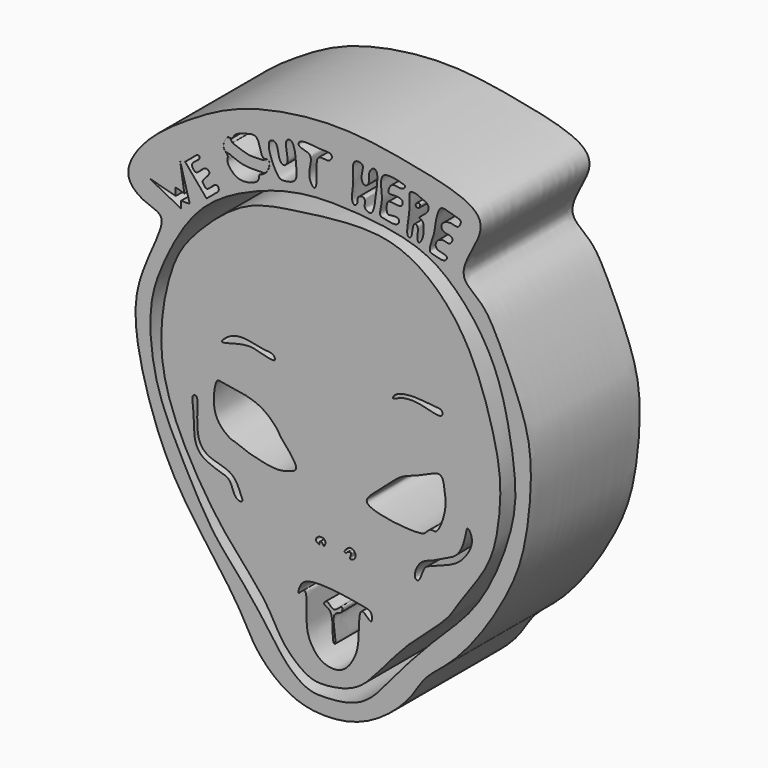
from build123d import *

# Parameters (mm, degrees)
F1_DEPTH = 12


# Not quite as in the source:
# - a feature names something its author has since deleted; it is built from what else it names


with BuildPart() as f1:
    # F0 (on Front) → F1 (new body)
    with BuildSketch(Plane.XZ):
        with BuildLine():
            add(Edge.make_bspline(
                [(-47.0166243613, 44.8620691895), (-45.595251877, 45.776944077), (-42.2741227464, 47.7877491265), (-34.0176381654, 49.1391279437), (-27.6370435065, 48.027277594), (-23.191439719, 47.1215840657), (-21.197445005, 46.0254771062), (-20.9193717284, 44.4684259144), (-22.5035572971, 42.0546528765), (-22.7690901071, 40.3377748917), (-20.8843213118, 39.2071538838), (-19.6447559897, 37.0583489704), (-17.633566432, 32.6179743092), (-16.4023527537, 28.7667152956), (-16.916817699, 22.3336429781), (-18.0728468976, 18.3576353556), (-20.7470243169, 13.731212027), (-23.6453545353, 10.2470769915), (-26.1614221001, 8.5326667329), (-27.2405305623, 6.2194756967), (-30.5742150796, 3.3267319265), (-34.1911424438, 2.4165036843), (-37.8655474923, 2.8581800799), (-40.9480017394, 5.5727937583), (-42.1845902774, 8.3976566392), (-45.0170046598, 12.252109148), (-47.5829757261, 15.6966068437), (-49.6990101842, 19.8737084463), (-51.4091567908, 25.4811818071), (-51.8436489228, 30.6040680499), (-49.3464398381, 35.1945462838), (-49.0787891391, 36.9579414452), (-50.8399233715, 37.2709356223), (-52.8928865029, 38.9279900141), (-50.646604664, 42.436379878), (-48.3189845132, 44.0237973006), (-47.0166243613, 44.8620691895)],
                knots=[0, 0, 0, 0, 0.0355770683, 0.0793528757, 0.1187531848, 0.1509720013, 0.1725011929, 0.1899685641, 0.2157418654, 0.2344161387, 0.2552668169, 0.2794632534, 0.3127171361, 0.3440503941, 0.3820044117, 0.4134842243, 0.4484589959, 0.4811195553, 0.5068947662, 0.5308536817, 0.5623016146, 0.5916301045, 0.620359809, 0.6502239744, 0.6771282332, 0.7101499943, 0.7419335424, 0.7747889469, 0.8115699797, 0.8464105758, 0.8808110455, 0.8982397629, 0.9169922383, 0.93908403, 0.96740182, 1, 1, 1, 1], degree=3))
        make_face()
        with BuildLine():
            add(Edge.make_bspline(
                [(-38.4240150452, 42.1812050045), (-37.0678788492, 42.5218744662), (-34.3867781007, 42.8088010896), (-28.3798473119, 42.3274214714), (-24.1902437, 40.8098863437), (-19.8961635432, 35.6901117013), (-18.6253817253, 30.528621672), (-18.0581329266, 27.0595758172), (-17.8633858275, 23.0739012141), (-20.7079995076, 15.7863490066), (-24.450016641, 12.3873464297), (-27.2230581422, 9.3965022394), (-29.0126764634, 7.3723433058), (-31.2995555124, 4.3586146755), (-34.6274425345, 4.0112345038), (-36.4516832364, 4.0578458846), (-38.3722620753, 5.6080571102), (-39.6856518206, 7.5759460913), (-42.1423981818, 10.8035289735), (-44.8206668482, 13.5361271115), (-47.6013889681, 18.7964344106), (-49.9213569734, 23.4284872311), (-50.5031038055, 29.324048), (-49.2168686424, 33.0878991596), (-46.6874092768, 37.918528947), (-43.0773019309, 40.6065854083), (-39.8897478434, 41.8130042257), (-38.4240150452, 42.1812050045)],
                knots=[0, 0, 0, 0, 0.0393324741, 0.0861492727, 0.1269776985, 0.1760073002, 0.2206521584, 0.2561939723, 0.2945424829, 0.3480010505, 0.3922375976, 0.4304492998, 0.4625965925, 0.4993837574, 0.5337407214, 0.5595497864, 0.5886036071, 0.6188415895, 0.6572680082, 0.6956866915, 0.7423767025, 0.7873017999, 0.8331769589, 0.8719791181, 0.9163532505, 0.9574888588, 1, 1, 1, 1], degree=3))
        make_face(mode=Mode.SUBTRACT)
        Polygon((-47.5117638707, 37.8683283925), (-50.2995289862, 39.3151417375), (-47.9881539941, 38.6976003647), (-47.9881539941, 39.3680743873), (-47.2294613719, 39.1387008131), (-47.5999861956, 41.5382944047), (-46.7530712485, 38.4858697653), (-47.5117638707, 38.4858697653), align=None, mode=Mode.SUBTRACT)
        with BuildLine():
            Line((-45.2709682286, 39.3857210875), (-47.1588820219, 41.6265167296))
            Line((-47.1588820219, 41.6265167296), (-46.1392381304, 42.4855864863))
            add(Edge.make_bspline(
                [(-46.1392381304, 42.4855864863), (-46.0465615658, 42.5054674734), (-45.8594185494, 42.5456134145), (-45.8520416375, 42.1577943123), (-46.6511050845, 41.7832702106), (-46.4903258591, 41.2952470764), (-46.1022131536, 40.9477511118), (-45.5256395853, 41.8046746664), (-45.067552008, 41.6403244999), (-44.9381597234, 41.3477459308), (-45.6719466599, 40.6847546609), (-45.5906592697, 40.4745039867), (-45.1946911115, 39.8798795628), (-44.5937516593, 40.8455123959), (-44.1630185636, 40.6303502121), (-44.1921356311, 40.3988699414), (-44.2067978835, 40.282305245)],
                knots=[0, 0, 0, 0, 0.052085804, 0.105177555, 0.2008801244, 0.2698978457, 0.3346360985, 0.4345195347, 0.5005230921, 0.55286709, 0.6548123539, 0.7045411848, 0.7779620534, 0.8784844899, 0.9388093918, 1, 1, 1, 1], degree=3))
            Line((-44.2067978835, 40.282305245), (-45.2709682286, 39.3857210875))
        make_face(mode=Mode.SUBTRACT)
        with BuildLine():
            add(Edge.make_bspline(
                [(-43.2456322014, 44.7879135609), (-43.1773507865, 44.7833628103), (-43.1203474246, 44.7420608165), (-43.0675894022, 44.7582378983)],
                knots=[0.9714162948, 0.9714162948, 0.9714162948, 0.9714162948, 1, 1, 1, 1], degree=3))
            add(Edge.make_bspline(
                [(-43.0675894022, 44.7582378983), (-42.9989112357, 44.7792965406), (-42.8691053132, 45.0293929425), (-42.6221246051, 45.3184155301), (-41.7475783885, 45.5732360318), (-40.5945532549, 45.8870759647), (-40.4806599693, 43.8436857931), (-39.9417733644, 44.2096012545), (-39.8331619799, 44.1647656262)],
                knots=[0, 0, 0, 0, 0.0372090608, 0.0785561522, 0.1434088997, 0.2074830467, 0.2888642065, 0.3329958717, 0.3329958717, 0.3329958717, 0.3329958717], degree=3))
            add(Edge.make_bspline(
                [(-39.8331619538, 44.1647656213), (-39.7602766999, 44.151206379), (-39.7284395126, 44.0661324711), (-39.7243966212, 43.9518775136)],
                knots=[0.2945540531, 0.2945540531, 0.2945540531, 0.2945540531, 0.3190794148, 0.3190794148, 0.3190794148, 0.3190794148], degree=3))
            add(Edge.make_bspline(
                [(-39.7243966212, 43.9518775136), (-39.7113465111, 43.832177882), (-39.7669607284, 43.3489257107), (-40.2487411874, 42.8370991823), (-40.6788729245, 42.8083932279), (-40.6142458833, 42.3132435515), (-41.0418230498, 41.9490622949), (-42.1032965277, 41.6892524188), (-42.908668964, 42.0081766665), (-43.5614733789, 42.8371202287), (-43.2981182226, 43.3150401101), (-43.5696992665, 43.5194752336), (-43.660394971, 43.6435321849)],
                knots=[0.3580242307, 0.3580242307, 0.3580242307, 0.3580242307, 0.3862259474, 0.4480160925, 0.4867681426, 0.5281473049, 0.5763905528, 0.6452541069, 0.7081336536, 0.7733064754, 0.8182050994, 0.8561222233, 0.8561222233, 0.8561222233, 0.8561222233], degree=3))
            add(Edge.make_bspline(
                [(-43.660394971, 43.6435321849), (-43.7865917542, 43.7698978255), (-43.8055004646, 44.0023963662), (-43.7281247793, 44.2474911359)],
                knots=[0.8330439372, 0.8330439372, 0.8330439372, 0.8330439372, 0.8755337844, 0.8755337844, 0.8755337844, 0.8755337844], degree=3))
            add(Edge.make_bspline(
                [(-43.7281247647, 44.2474911871), (-43.6928008455, 44.3719700456), (-43.6167159272, 44.5325123333), (-43.5244744487, 44.6411680027), (-43.4995404875, 44.6661314575)],
                knots=[0.9030772587, 0.9030772587, 0.9030772587, 0.9030772587, 0.9295678201, 0.9390671556, 0.9390671556, 0.9390671556, 0.9390671556], degree=3))
            add(Edge.make_bspline(
                [(-43.4995404875, 44.6661314575), (-43.413944485, 44.7634769709), (-43.3218092162, 44.8182348636), (-43.2456322014, 44.7879135609)],
                knots=[0.9021251558, 0.9021251558, 0.9021251558, 0.9021251558, 0.9263325769, 0.9263325769, 0.9263325769, 0.9263325769], degree=3))
        make_face(mode=Mode.SUBTRACT)
        with BuildLine():
            add(Edge.make_bspline(
                [(-39.7415310144, 45.5790273845), (-39.9445700993, 45.0899409234), (-39.076085851, 43.0825175549), (-38.545065207, 42.9345275653), (-37.3027436398, 43.1510735203), (-37.3185511717, 44.2461944438), (-37.5140119737, 46.4624062707), (-38.2487786003, 46.3009786949), (-38.293273575, 45.7319646594), (-38.1168506677, 44.9346337394), (-38.1015809471, 44.4595086479), (-38.4929023876, 44.0319639145), (-38.9845528625, 44.6133548632), (-38.9777428469, 45.9043106405), (-39.6454047044, 45.8105792398), (-39.7415310144, 45.5790273845)],
                knots=[0, 0, 0, 0, 0.1312235203, 0.1949314617, 0.2786049754, 0.3642703204, 0.4835971299, 0.5359197008, 0.5955830633, 0.6724402957, 0.7304539966, 0.7835419666, 0.8478830825, 0.937873869, 1, 1, 1, 1], degree=3))
        make_face(mode=Mode.SUBTRACT)
        with BuildLine():
            add(Edge.make_bspline(
                [(-37.0067022741, 46.4965216815), (-37.1571867188, 46.4032603575), (-37.2607087523, 45.9546746534), (-35.8664058245, 45.9719520528), (-36.2034844106, 44.6782350919), (-36.2534624056, 43.8823964905), (-35.7949926392, 43.1371333176), (-35.5293838928, 43.6181235302), (-35.6002153106, 44.6731321226), (-35.5539823511, 45.8598584987), (-35.0234132886, 45.8590436672), (-34.4226287785, 45.7488078966), (-34.1439951194, 46.1976469241), (-34.3890364819, 46.5292450078), (-35.2685805871, 46.416806358), (-36.6860703352, 46.6952303203), (-37.0067022741, 46.4965216815)],
                knots=[0, 0, 0, 0, 0.0521113404, 0.1354071728, 0.2208503286, 0.3017367921, 0.3683065166, 0.4148283754, 0.5059676652, 0.5926154433, 0.6458894091, 0.7103345129, 0.7641496111, 0.8087478712, 0.8889681911, 1, 1, 1, 1], degree=3))
        make_face(mode=Mode.SUBTRACT)
        with BuildLine():
            add(Edge.make_bspline(
                [(-32.207518816, 46.4965216815), (-32.4701286429, 46.2505183013), (-32.173270173, 44.9124336744), (-32.5962911284, 43.5742952887), (-32.1932073961, 42.9676291969), (-31.8929098487, 43.4543410085), (-31.996544244, 43.8961039159), (-31.5094488704, 44.0397093737), (-31.2521699762, 43.8771410453), (-31.3619723855, 43.3056399132), (-31.2590036508, 43.0726525174), (-30.7426859742, 42.8393878073), (-30.4429532561, 43.4965999427), (-30.3413501835, 44.6178538877), (-30.0945805073, 46.2277720064), (-30.5166045943, 46.6143201902), (-31.0577042812, 46.1268052258), (-30.8541406305, 45.1759822328), (-31.2721103899, 44.8820149808), (-31.627975952, 45.1482875767), (-31.5915898163, 45.8325901117), (-31.3387005167, 46.6151939086), (-32.0355516895, 46.657614261), (-32.207518816, 46.4965216815)],
                knots=[0, 0, 0, 0, 0.0751043617, 0.1497401555, 0.1896895528, 0.2277881385, 0.2668540958, 0.3051825112, 0.335001314, 0.3792866057, 0.4098807216, 0.4495249579, 0.4945890761, 0.5626496753, 0.6393918126, 0.6760162216, 0.7211153381, 0.7795538627, 0.8162648223, 0.8511361484, 0.9016374869, 0.9508187435, 1, 1, 1, 1], degree=3))
        make_face(mode=Mode.SUBTRACT)
        with BuildLine():
            add(Edge.make_bspline(
                [(-29.6667721123, 46.2495014071), (-30.0210563778, 45.96228624), (-29.6812809427, 44.4997162614), (-29.93374072, 43.6192435306), (-30.016369393, 42.9674318885), (-29.5685790665, 42.9306325776), (-28.6907209596, 42.6813379227), (-28.2151086076, 42.9880501216), (-28.3263866047, 43.4453699199), (-28.9378029318, 43.3816277828), (-29.3714624213, 43.3000493275), (-29.3923785748, 43.8555947667), (-29.3640407308, 44.5615161698), (-28.3345185746, 44.2651888702), (-27.9587394284, 44.4455776297), (-27.9332912344, 45.0204344511), (-28.8233305201, 45.0013130292), (-29.2876999038, 44.9747414355), (-29.1849051034, 45.4108113406), (-28.8973826226, 45.9707927506), (-28.0431771095, 45.5939056842), (-27.6601840592, 46.0609613156), (-28.053211092, 46.1981489551), (-29.3166937662, 46.533306872), (-29.6667721123, 46.2495014071)],
                knots=[0, 0, 0, 0, 0.0767138938, 0.1372744162, 0.1788486331, 0.2142028463, 0.2711139713, 0.3112350505, 0.3443083771, 0.3887964801, 0.4239550965, 0.4643824731, 0.507676459, 0.5632379223, 0.5992626883, 0.6353483812, 0.688369378, 0.7245560158, 0.7588973557, 0.801810777, 0.854541806, 0.8913362498, 0.9241968225, 1, 1, 1, 1], degree=3))
        make_face(mode=Mode.SUBTRACT)
        with BuildLine():
            add(Edge.make_bspline(
                [(-27.2848233581, 45.7378253341), (-27.4687439624, 45.5785716873), (-27.2113067326, 44.4378192887), (-27.7260398826, 42.5317109866), (-27.4044327738, 42.0999633247), (-27.1297524026, 42.3277276756), (-27.1073580545, 43.2399296677), (-26.8206953751, 43.4822950774), (-26.5517452822, 43.1632308338), (-26.7337842952, 42.3612686371), (-26.5509429247, 41.8873142899), (-26.1400327053, 42.5601783326), (-26.1074559891, 43.243005087), (-26.1443361495, 43.8974673767), (-26.7478155867, 43.9845326778), (-25.6395283889, 44.5723025675), (-25.6661765194, 45.3660941409), (-26.3457924334, 45.5461039106), (-26.6716722767, 45.7565012723), (-27.1606282974, 45.8453636733), (-27.2848233581, 45.7378253341)],
                knots=[0, 0, 0, 0, 0.0796896171, 0.1823733062, 0.2236935715, 0.2585851936, 0.3272956199, 0.3639728173, 0.4024973082, 0.4690927292, 0.5077950583, 0.5612885755, 0.6246793841, 0.6793128134, 0.7171383344, 0.7859620856, 0.8430817502, 0.8985494075, 0.946188428, 1, 1, 1, 1], degree=3))
        make_face(mode=Mode.SUBTRACT)
        with BuildLine():
            add(Edge.make_bspline(
                [(-24.7264355421, 45.226149261), (-24.9058755261, 44.94221811), (-25.1599766356, 43.7401625597), (-25.1649704713, 43.1365384494), (-25.8050755898, 41.6079233381), (-25.146835507, 41.5520256673), (-24.2793316895, 41.2177853045), (-23.9293729085, 41.7821547576), (-24.5175208785, 41.9413488885), (-24.918051452, 42.0009601435), (-25.1296276043, 42.3127704059), (-24.9288606955, 42.8627909619), (-24.2990481815, 42.9786894434), (-23.8765793087, 42.745454019), (-23.5852269645, 43.0783860353), (-23.5559078587, 43.3377240835), (-23.8279825095, 43.5515002028), (-24.3083673277, 43.5000246673), (-24.6882723072, 43.9583211724), (-24.3275653077, 44.446070451), (-23.6746153675, 44.5253964681), (-23.1694062802, 44.3042487984), (-22.9264211164, 44.5335595521), (-22.7523161869, 44.9822670441), (-23.3278079497, 45.1401544908), (-24.354142761, 45.4734799772), (-24.6308713211, 45.3773622664), (-24.7264355421, 45.226149261)],
                knots=[0, 0, 0, 0, 0.0659449797, 0.1151764838, 0.1787265422, 0.2158169585, 0.2675599616, 0.3014304502, 0.3391521643, 0.3748581597, 0.4053153803, 0.444007476, 0.4858305884, 0.5217508393, 0.5547369265, 0.5810316163, 0.6105230742, 0.6479934645, 0.6854102995, 0.7235697432, 0.7675628444, 0.806399821, 0.8358913541, 0.8689554225, 0.9076111196, 0.9648797304, 1, 1, 1, 1], degree=3))
        make_face(mode=Mode.SUBTRACT)
    extrude(amount=F1_DEPTH)


with BuildPart() as f1b:
    # F0 (on Front) → F1, piece 2 (new body)
    with BuildSketch(Plane.XZ):
        with BuildLine():
            add(Edge.make_bspline(
                [(-26.7555024475, 45.0497083366), (-26.8285066461, 44.9759407264), (-26.8704578621, 44.7030808747), (-26.4747340143, 44.6944044468), (-26.4170097172, 44.9799385502), (-26.4860008388, 45.1397857044), (-26.6867099293, 45.1192202244), (-26.7555024475, 45.0497083366)],
                knots=[0, 0, 0, 0, 0.2200516962, 0.4325267283, 0.6370433084, 0.7926432918, 1, 1, 1, 1], degree=3))
        make_face()
    extrude(amount=F1_DEPTH)


with BuildPart() as f1c:
    # F0 (on Front) → F1, piece 3 (new body)
    with BuildSketch(Plane.XZ):
        with BuildLine():
            add(Edge.make_bspline(
                [(-38.1272435188, 40.888544172), (-36.7406212912, 41.1046865303), (-33.8662895674, 41.5051343883), (-29.5292426681, 41.6891083312), (-25.791418619, 40.0401086633), (-21.9906255692, 35.9334700559), (-19.8421048002, 29.3072658946), (-19.1944981493, 25.4687381622), (-19.6052665652, 21.3432693388), (-20.511499701, 18.5528459974), (-23.0468525687, 15.2907578033), (-23.7516065277, 13.8820997312), (-26.0685601156, 11.7518112154), (-27.6253899824, 10.4821181902), (-30.0219070772, 7.66224875), (-31.9626341834, 5.4064944246), (-34.9487489928, 4.9034306974), (-36.4872309338, 5.1245361219), (-38.7467987259, 7.0858517176), (-39.7236074655, 9.6029975232), (-42.8919618661, 12.9969950274), (-45.0346138382, 15.731519662), (-47.930315631, 20.5751612576), (-49.8239849539, 26.4201105608), (-48.4989124156, 33.3692980656), (-46.4564007549, 36.3124991162), (-42.2731275007, 40.1932001918), (-39.4857085019, 40.6767908774), (-38.1272435188, 40.888544172)],
                knots=[0, 0, 0, 0, 0.0409164396, 0.0814310005, 0.1201087028, 0.1663081448, 0.2179277749, 0.2572082629, 0.2960953076, 0.3306077275, 0.3695390796, 0.3951006857, 0.428766107, 0.4576433886, 0.4949945718, 0.5292802757, 0.5620294647, 0.586335007, 0.618793739, 0.6517010038, 0.6932724263, 0.7305608375, 0.7764961678, 0.8258465613, 0.8766493403, 0.9142572465, 0.9599144242, 1, 1, 1, 1], degree=3))
        make_face()
        with BuildLine():
            add(Edge.make_bspline(
                [(-46.4555434883, 23.7064473331), (-46.5899280144, 23.5317670701), (-46.3406758796, 22.4132157769), (-46.4589206692, 20.5242485113), (-45.8967955288, 19.3061188112), (-44.9193762607, 18.834884362), (-44.0274589029, 18.5121077394), (-43.065295873, 18.3066418616), (-42.8646787336, 16.8568714151), (-41.9789106542, 16.7927120381), (-42.2896913837, 17.4577387881), (-42.8258531891, 18.9082093664), (-44.669927893, 19.1798060701), (-46.2457600919, 20.070409075), (-46.0395832028, 22.9518581114), (-46.0830674983, 23.8253115945), (-46.3924582176, 23.7884489742), (-46.4555434883, 23.7064473331)],
                knots=[0, 0, 0, 0, 0.068165907, 0.1575936194, 0.2275087785, 0.2910430575, 0.3526710202, 0.4113738391, 0.4826614156, 0.527407917, 0.57176196, 0.6478203645, 0.7307946128, 0.8104269733, 0.9149878316, 0.9680002987, 1, 1, 1, 1], degree=3))
        make_face(mode=Mode.SUBTRACT)
        with BuildLine():
            add(Edge.make_bspline(
                [(-35.3057868779, 15.7720558345), (-35.2747962391, 15.7970027785), (-35.3787016938, 15.9959797076), (-35.0754892037, 16.0932912157), (-34.9546164861, 15.6504358261), (-34.7463777486, 16.0079886816), (-34.8494063602, 16.3967590795), (-35.4336213459, 16.4275362475), (-35.7594598933, 15.957110136), (-35.3481060186, 15.7379896366), (-35.3057868779, 15.7720558345)],
                knots=[0, 0, 0, 0, 0.0978925494, 0.1957885511, 0.3184834077, 0.429832325, 0.5627614581, 0.720847005, 0.8663232272, 1, 1, 1, 1], degree=3))
        make_face(mode=Mode.SUBTRACT)
        with BuildLine():
            add(Edge.make_bspline(
                [(-44.3144850433, 25.5641229451), (-44.2269449166, 25.6460537274), (-43.8989794184, 25.5046259957), (-42.0176616083, 25.3689401665), (-40.0573742202, 24.7111933062), (-38.8420198577, 23.3001075192), (-38.8109854799, 22.9949500489), (-36.8686356086, 21.011279129), (-37.9945894278, 20.5511523569), (-39.258180312, 20.2383239766), (-41.0793645966, 20.7440027837), (-41.4127044297, 20.7792311061), (-42.7542232392, 21.351006314), (-43.0918354547, 21.33055698), (-44.3826880087, 22.2531710023), (-44.7606111392, 23.9030472172), (-44.4967314704, 25.3935543966), (-44.3144850433, 25.5641229451)],
                knots=[0, 0, 0, 0, 0.0363374958, 0.1186428758, 0.2099461396, 0.2872872136, 0.3260844703, 0.4182766599, 0.4695745224, 0.5424252901, 0.6229970177, 0.662764139, 0.7331468586, 0.7709581179, 0.8419465743, 0.9243503633, 1, 1, 1, 1], degree=3))
        make_face(mode=Mode.SUBTRACT)
        with BuildLine():
            add(Edge.make_bspline(
                [(-37.1057540178, 11.7599451914), (-37.0049982917, 12.0605422822), (-36.5888063201, 12.8779425142), (-33.1688041406, 12.5558638289), (-31.27051169, 12.1854458871), (-30.6602546419, 12.0322500811), (-30.640019884, 10.854364602), (-31.3910855569, 11.8950973372), (-31.8672030243, 11.685842411), (-31.796807077, 9.441031982), (-32.0929242654, 8.0545021687), (-33.2147988822, 6.3435576837), (-35.0863235167, 6.5394786178), (-36.0312944197, 7.6636769371), (-36.6182555642, 9.0120796534), (-36.2603824077, 12.4726486524), (-37.2695983597, 11.1427738505), (-37.1672669835, 11.5764259094), (-37.1057540178, 11.7599451914)],
                knots=[0, 0, 0, 0, 0.0550543234, 0.1562731093, 0.2356683001, 0.2761318952, 0.320199333, 0.3706569874, 0.4007978588, 0.4812027976, 0.5520249182, 0.6266334881, 0.6972568905, 0.7613842181, 0.8348809556, 0.9225631544, 0.9663884641, 1, 1, 1, 1], degree=3))
        make_face(mode=Mode.SUBTRACT)
        with BuildLine():
            add(Edge.make_bspline(
                [(-33.0423377454, 16.0496905446), (-32.9779016491, 16.1387469259), (-32.7975416629, 16.3310949739), (-32.528031786, 16.4344898129), (-32.0762671914, 16.1582293479), (-32.1194676216, 15.6174777227), (-32.6850639823, 15.4067602116), (-32.5630015134, 15.7750668037), (-32.4503700068, 16.1031963101), (-32.8613944593, 16.0293919818), (-32.9482037479, 15.8318068466), (-33.1367487814, 15.8949275611), (-33.0840688531, 15.9920144648), (-33.0423377454, 16.0496905446)],
                knots=[0, 0, 0, 0, 0.1032998952, 0.1914866304, 0.3060813229, 0.4225136692, 0.5299909531, 0.6176885623, 0.7053860165, 0.7972620908, 0.8738970962, 0.933099314, 1, 1, 1, 1], degree=3))
        make_face(mode=Mode.SUBTRACT)
        with BuildLine():
            add(Edge.make_bspline(
                [(-30.2641056478, 21.5348154306), (-29.5199805948, 22.1818080565), (-28.2636449547, 23.4415455938), (-27.0479444509, 23.7396999675), (-25.5785656633, 24.427008298), (-24.4314642, 24.8859257722), (-24.2392867321, 23.2651322147), (-24.0869163786, 22.1040150417), (-24.8639084235, 19.8692900159), (-25.4578913804, 20.2212148564), (-25.8956569274, 19.8012190411), (-26.2597939993, 19.2810290401), (-32.3117909091, 19.90310256), (-30.8062287174, 21.063456985), (-30.2641056478, 21.5348154306)],
                knots=[0, 0, 0, 0, 0.1162111221, 0.1942666454, 0.2846525167, 0.3512345559, 0.4289440158, 0.5133930902, 0.6121827495, 0.6577291113, 0.7062407597, 0.7631534675, 0.9153358297, 1, 1, 1, 1], degree=3))
        make_face(mode=Mode.SUBTRACT)
        with BuildLine():
            add(Edge.make_bspline(
                [(-25.3212396055, 17.7748352289), (-24.9676944516, 17.9160229961), (-24.2727431069, 18.3239727686), (-22.9451252469, 18.7923282808), (-22.4188969378, 20.5473446361), (-22.2923732628, 21.5671626388), (-21.6102030472, 20.3991540326), (-22.4093954121, 18.9172532605), (-23.4311556056, 17.9763719059), (-25.5573627959, 17.2818752417), (-26.144019628, 16.9946349443), (-26.4607700659, 15.6966912745), (-26.9169866373, 15.8320713863), (-26.9310945462, 16.4260145248), (-26.3720083665, 17.4717055744), (-25.6587946028, 17.6400331086), (-25.3212396055, 17.7748352289)],
                knots=[0, 0, 0, 0, 0.0751115916, 0.1549721077, 0.2491243654, 0.3033097825, 0.365975401, 0.453821416, 0.5382705362, 0.6394680075, 0.696846906, 0.7707924803, 0.8056396664, 0.8550211642, 0.9282855589, 1, 1, 1, 1], degree=3))
        make_face(mode=Mode.SUBTRACT)
        with BuildLine():
            add(Edge.make_bspline(
                [(-43.295647949, 29.3089430779), (-42.8533668426, 29.5687375343), (-41.8812970789, 29.7344024537), (-40.3670472119, 29.2366956298), (-39.3598184574, 29.323158348), (-39.069740225, 28.5296239833), (-40.7022295263, 29.0395236181), (-41.5403547332, 29.2011488859), (-42.7412697985, 28.9766185549), (-44.311922337, 28.4675838982), (-43.6341892506, 29.1100850391), (-43.295647949, 29.3089430779)],
                knots=[0, 0, 0, 0, 0.1294957123, 0.2660827668, 0.3700032985, 0.4355704696, 0.5596605547, 0.6661495499, 0.7903929518, 0.9008783184, 1, 1, 1, 1], degree=3))
        make_face(mode=Mode.SUBTRACT)
        with BuildLine():
            add(Edge.make_bspline(
                [(-26.1910948902, 29.8933982849), (-25.7884778095, 29.8573157418), (-25.1921393095, 29.7575360504), (-24.4486270312, 29.7938061735), (-24.4167450158, 28.9079892397), (-26.4974449564, 29.7182118941), (-28.1047954597, 29.5921381056), (-28.9551655603, 29.0511984752), (-28.6841038606, 29.6438437021), (-27.7125210673, 29.9606673747), (-26.6747895665, 29.9367470022), (-26.1910948902, 29.8933982849)],
                knots=[0, 0, 0, 0, 0.1179642045, 0.2066507974, 0.2785609634, 0.4335722394, 0.5886895171, 0.6787306602, 0.7435513659, 0.8582805836, 1, 1, 1, 1], degree=3))
        make_face(mode=Mode.SUBTRACT)
    extrude(amount=F1_DEPTH)


with BuildPart() as f1d:
    # F0 (on Front) → F1, piece 4 (new body)
    with BuildSketch(Plane.XZ):
        with BuildLine():
            add(Edge.make_bspline(
                [(-34.6550643444, 11.5475412458), (-34.4653946882, 11.5328117594), (-34.0783605325, 10.7112189946), (-33.2516490737, 11.8906130693), (-33.2736457659, 10.9161406027), (-34.4678184522, 11.0798291352), (-33.6772937073, 8.4032366118), (-34.2925796989, 8.5147280105), (-33.9251676953, 11.1415367911), (-35.0965581754, 11.1404148054), (-34.7860746095, 11.5577153241), (-34.6550643444, 11.5475412458)],
                knots=[0, 0, 0, 0, 0.1069803906, 0.2174780328, 0.2972564818, 0.4042368724, 0.5874949913, 0.6355807008, 0.8244173844, 0.9261055795, 1, 1, 1, 1], degree=3))
        make_face()
    extrude(amount=F1_DEPTH)


with BuildPart() as f1e:
    # F0 (on Front) → F1, piece 5 (new body)
    with BuildSketch(Plane.XZ):
        with BuildLine():
            add(Edge.make_bspline(
                [(-39.8331619553, 44.164765616), (-39.7715652756, 44.1393380076), (-39.7359782848, 44.0581081015), (-39.7243966212, 43.9518775136)],
                knots=[0.3329958751, 0.3329958751, 0.3329958751, 0.3329958751, 0.3580242307, 0.3580242307, 0.3580242307, 0.3580242307], degree=3))
            add(Edge.make_bspline(
                [(-40.3725957474, 43.9845794257), (-40.1962351414, 44.0067321434), (-39.9562057475, 44.1876560991), (-39.8331619799, 44.1647656262)],
                knots=[0.2531507163, 0.2531507163, 0.2531507163, 0.2531507163, 0.2945540502, 0.2945540502, 0.2945540502, 0.2945540502], degree=3))
            add(Edge.make_bspline(
                [(-40.4327120387, 43.9840486534), (-40.4137848767, 43.9815531998), (-40.3936437471, 43.981935579), (-40.3725957474, 43.9845794257)],
                knots=[0.2482093783, 0.2482093783, 0.2482093783, 0.2482093783, 0.2531507163, 0.2531507163, 0.2531507163, 0.2531507163], degree=3))
            add(Edge.make_bspline(
                [(-42.9815426469, 44.4485805929), (-42.5014464873, 44.2710513108), (-41.7251128647, 43.9862850964), (-41.2081885689, 43.9591487918), (-40.7077852535, 43.9809524179), (-40.4327120387, 43.9840486534)],
                knots=[0, 0, 0, 0, 0.417243017, 0.6754963365, 0.9779862, 0.9779862, 0.9779862, 0.9779862], degree=3))
            add(Edge.make_bspline(
                [(-43.2456322014, 44.7879135609), (-43.1224785404, 44.7388937949), (-43.041034105, 44.4675071357), (-42.9815426469, 44.4485805929)],
                knots=[0.9263325769, 0.9263325769, 0.9263325769, 0.9263325769, 0.9654681683, 0.9654681683, 0.9654681683, 0.9654681683], degree=3))
            add(Edge.make_bspline(
                [(-43.4995404875, 44.6661314575), (-43.4146301088, 44.7511422743), (-43.3229085721, 44.7930637981), (-43.2456322014, 44.7879135609)],
                knots=[0.9390671556, 0.9390671556, 0.9390671556, 0.9390671556, 0.9714162948, 0.9714162948, 0.9714162948, 0.9714162948], degree=3))
            add(Edge.make_bspline(
                [(-43.7281247633, 44.2474911867), (-43.6797008255, 44.4008785443), (-43.5935659867, 44.5591993554), (-43.4995404875, 44.6661314575)],
                knots=[0.8755337873, 0.8755337873, 0.8755337873, 0.8755337873, 0.9021251558, 0.9021251558, 0.9021251558, 0.9021251558], degree=3))
            add(Edge.make_bspline(
                [(-43.660394971, 43.6435321849), (-43.6905558498, 43.6847873545), (-43.7890131597, 43.8509569701), (-43.7739231245, 44.0861011814), (-43.7281247647, 44.2474911871)],
                knots=[0.8561222233, 0.8561222233, 0.8561222233, 0.8561222233, 0.8687315721, 0.9030772587, 0.9030772587, 0.9030772587, 0.9030772587], degree=3))
            add(Edge.make_bspline(
                [(-43.0938266218, 43.4255301952), (-43.1610895627, 43.5294483502), (-43.4761459895, 43.4953317943), (-43.6420690401, 43.625181733), (-43.660394971, 43.6435321849)],
                knots=[0.7833175872, 0.7833175872, 0.7833175872, 0.7833175872, 0.8268736848, 0.8330439372, 0.8330439372, 0.8330439372, 0.8330439372], degree=3))
            add(Edge.make_bspline(
                [(-43.0938266218, 43.4255301952), (-42.7458113345, 43.2810234466), (-42.0117572102, 42.9762213914), (-41.0856291904, 43.0008582962), (-40.5985787511, 43.0138148367)],
                knots=[0, 0, 0, 0, 0.4741003091, 1, 1, 1, 1], degree=3))
            add(Edge.make_bspline(
                [(-39.7243966212, 43.9518775136), (-39.7215679773, 43.8719380448), (-39.7649489532, 43.492664338), (-40.0655413229, 42.899002436), (-40.4787087595, 43.0427761639), (-40.5985787511, 43.0138148367)],
                knots=[0.3190794148, 0.3190794148, 0.3190794148, 0.3190794148, 0.3362387962, 0.3881497741, 0.4281919664, 0.4281919664, 0.4281919664, 0.4281919664], degree=3))
        make_face()
        with BuildLine():
            add(Edge.make_bspline(
                [(-40.4327120387, 43.9840486534), (-40.4137848767, 43.9815531998), (-40.3936437471, 43.981935579), (-40.3725957474, 43.9845794257)],
                knots=[0.2482093783, 0.2482093783, 0.2482093783, 0.2482093783, 0.2531507163, 0.2531507163, 0.2531507163, 0.2531507163], degree=3))
            add(Edge.make_bspline(
                [(-40.4327120387, 43.9840486534), (-40.4126934944, 43.984273983), (-40.3926477625, 43.9844534173), (-40.3725957474, 43.9845794257)],
                knots=[0.9779862, 0.9779862, 0.9779862, 0.9779862, 1, 1, 1, 1], degree=3))
        make_face()
    extrude(amount=F1_DEPTH)


solid = Compound([f1.part, f1b.part, f1c.part, f1d.part, f1e.part])
